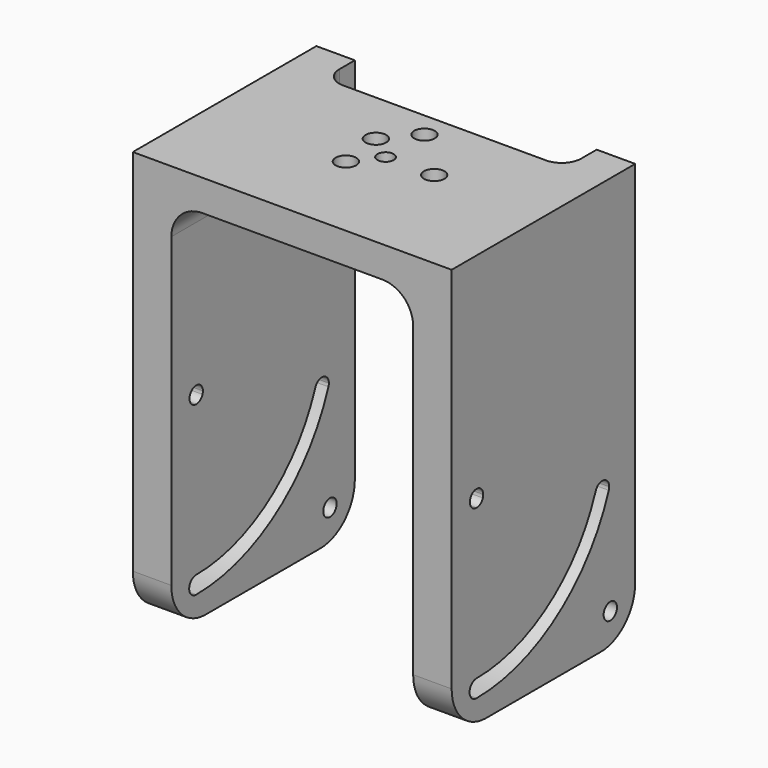
from build123d import *

# Parameters (mm, degrees)
F0_W     = 59
F0_H     = 8
F0_H_2   = 98
F0_R     = 2.15
F1_DEPTH = 82
F2_W     = 62.2
F2_H     = 98
F3_DEPTH = 25
F4_DEPTH = 125.3
F5_R     = 2.1
F5_R_2   = 2.65
F5_W     = 62.2
F5_H     = 10
F6_DEPTH = 20.8
F7_R     = 7.9669047558
F8_R     = 11.1053823869
F9_R     = 5


with BuildPart() as f1:
    # F0 (on Right) → F1 (new body)
    with BuildSketch(Plane.YZ):
        with Locations((21.5, 62.4624560177)):
            Rectangle(F0_W, F0_H)
        with Locations((21.5, 9.4624560177)):
            Rectangle(F0_W, F0_H_2)
        with BuildLine():
            ThreePointArc((0, -33.7875439823), (-2.25, -31.5375439823), (0, -29.2875439823))
            Line((0, -29.2875439823), (0, 9.3124560177))
            ThreePointArc((0, 9.3124560177), (-1.5202795796, 12.9827355973), (2.15, 11.4624560177))
            ThreePointArc((2.15, 11.4624560177), (2.117336669, 11.0891124357), (2.0203391347, 10.7271127096))
            Line((2.0203391347, 10.7271127096), (38.292474297, -2.4748648228))
            ThreePointArc((38.292474297, -2.4748648228), (40.7974910935, -1.028592701), (42.6567826938, -3.2444101453))
            ThreePointArc((42.6567826938, -3.2444101453), (42.6226001381, -3.635118545), (42.5210910906, -4.0139554678))
            ThreePointArc((42.5210910906, -4.0139554678), (25.9543337449, -25.6041739863), (0, -33.7875439823))
        make_face(mode=Mode.SUBTRACT)
        with Locations((43, -31.5375439823)):
            Circle(F0_R, mode=Mode.SUBTRACT)
        with BuildLine():
            Line((0, 9.3124560177), (0, -29.2875439823))
            ThreePointArc((0, -29.2875439823), (23.3732397813, -21.917989787), (38.292474297, -2.4748648228))
            Line((38.292474297, -2.4748648228), (2.0203391347, 10.7271127096))
            ThreePointArc((2.0203391347, 10.7271127096), (1.2331893382, 9.7012791225), (0, 9.3124560177))
        make_face()
    extrude(amount=F1_DEPTH)

    # F2 (on face) → F3 (join)
    with BuildSketch(Plane.XZ.offset(8)):
        with Locations((41, 9.4624560177)):
            Rectangle(F2_W, F2_H)
    extrude(amount=F3_DEPTH)

    # F4 (cut): a face of the model
    f4_faces = [f1.faces().sort_by_distance(p)[0] for p in [
        (41, -33, 9.4624560177),
    ]]
    extrude(f4_faces, amount=-F4_DEPTH, mode=Mode.SUBTRACT)

    # F5 (on face) → F6 (cut)
    with BuildSketch(Plane(origin=(0, 0, 58.4624560177), x_dir=(1, 0, 0), z_dir=(0, 0, -1))):
        with Locations((41, -22)):
            Circle(F5_R)
        with Locations((53.5, -22)):
            Circle(F5_R_2)
        with Locations((34.5, -27)):
            Circle(F5_R_2)
        with Locations((36, -15.5)):
            Circle(F5_R_2)
        with Locations((41, -34.5)):
            Circle(F5_R_2)
        with Locations((41, -46)):
            Rectangle(F5_W, F5_H)
    extrude(amount=-F6_DEPTH, mode=Mode.SUBTRACT)

    # F7
    f7_edges = [f1.edges().sort_by_distance(p)[0] for p in [
        (9.9, 16.5, 58.462456),
        (72.1, 16.5, 58.462456),
    ]]
    fillet(f7_edges, radius=F7_R)

    # F8
    f8_edges = [f1.edges().sort_by_distance(p)[0] for p in [
        (4.95, -8, -39.537544),
        (4.95, 51, -39.537544),
        (77.05, 51, -39.537544),
        (77.05, -8, -39.537544),
    ]]
    fillet(f8_edges, radius=F8_R)

    # F9
    f9_edges = [f1.edges().sort_by_distance(p)[0] for p in [
        (9.9, 41, 62.462456),
        (72.1, 41, 62.462456),
    ]]
    fillet(f9_edges, radius=F9_R)


solid = f1.part
